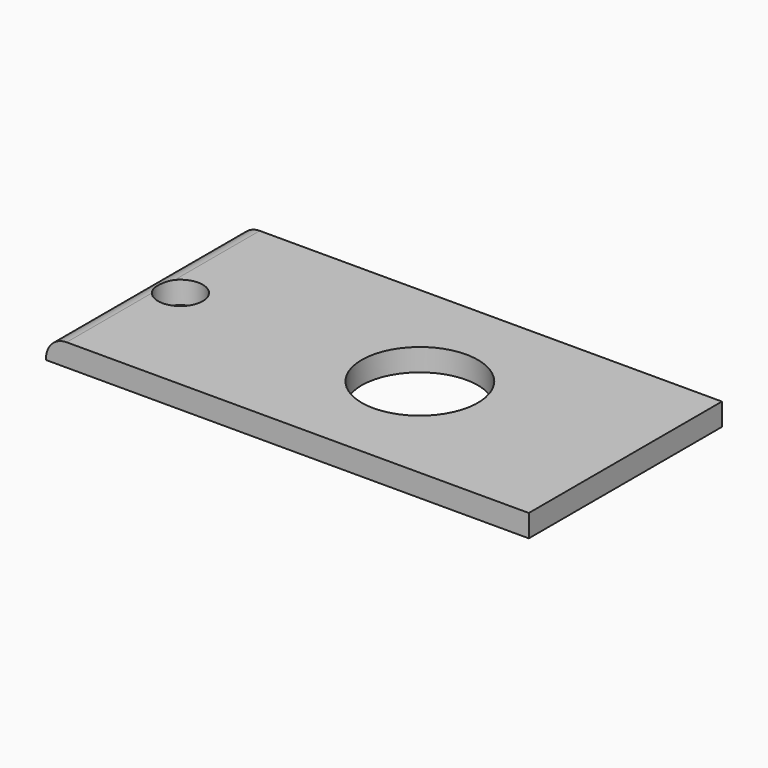
from build123d import *

# Parameters (mm, degrees)
F1_DEPTH    = 6.35
F2_T1_DEPTH = 97.79


# Not quite as in the source:
# - a fillet or chamfer that OpenCascade refuses, or shapes differently, is made with other operations: its cross-section is extruded or revolved along the edge and cut away or added


with BuildPart() as f1:
    # F0 (on Top) → F1 (new body)
    with BuildSketch(Plane.XY):
        with BuildLine():
            Line((-77.5854553002, 19.2668606828), (-77.5854553002, -15.0231393172))
            Line((-77.5854553002, -15.0231393172), (59.5745446998, -15.0231393172))
            Line((59.5745446998, -15.0231393172), (59.5745446998, 19.2668606828))
            Line((59.5745446998, 19.2668606828), (17.687636208, 19.2668606828))
            ThreePointArc((17.687636208, 19.2668606828), (1.177636208, 2.7568606828), (-15.332363792, 19.2668606828))
            Line((-15.332363792, 19.2668606828), (-60.4981811881, 19.2668606828))
            ThreePointArc((-60.4981811881, 19.2668606828), (-66.8481811881, 12.9168606828), (-73.1981811881, 19.2668606828))
            Line((-73.1981811881, 19.2668606828), (-77.5854553002, 19.2668606828))
        make_face()
        with BuildLine():
            Line((-77.5854553002, 53.5568606828), (-77.5854553002, 19.2668606828))
            Line((-77.5854553002, 19.2668606828), (-73.1981811881, 19.2668606828))
            ThreePointArc((-73.1981811881, 19.2668606828), (-66.8481811881, 25.6168606828), (-60.4981811881, 19.2668606828))
            Line((-60.4981811881, 19.2668606828), (-15.332363792, 19.2668606828))
            ThreePointArc((-15.332363792, 19.2668606828), (1.177636208, 35.7768606828), (17.687636208, 19.2668606828))
            Line((17.687636208, 19.2668606828), (59.5745446998, 19.2668606828))
            Line((59.5745446998, 19.2668606828), (59.5745446998, 53.5568606828))
            Line((59.5745446998, 53.5568606828), (-77.5854553002, 53.5568606828))
        make_face()
    extrude(amount=F1_DEPTH)

    # F2: fillet of radius 5.842 on 1 edges, made by hand

    # F2_s2 → F2_t1 (cut)
    with BuildSketch(Plane.XZ.offset(-68.1618606828)):
        with BuildLine():
            ThreePointArc((-77.5854553002, 0.508), (-75.8743731159, 4.6389178157), (-71.7434553002, 6.35))
            Line((-71.7434553002, 6.35), (-77.5854553002, 6.35))
            Line((-77.5854553002, 6.35), (-77.5854553002, 0.508))
        make_face()
    extrude(amount=F2_T1_DEPTH, mode=Mode.SUBTRACT)


solid = f1.part
